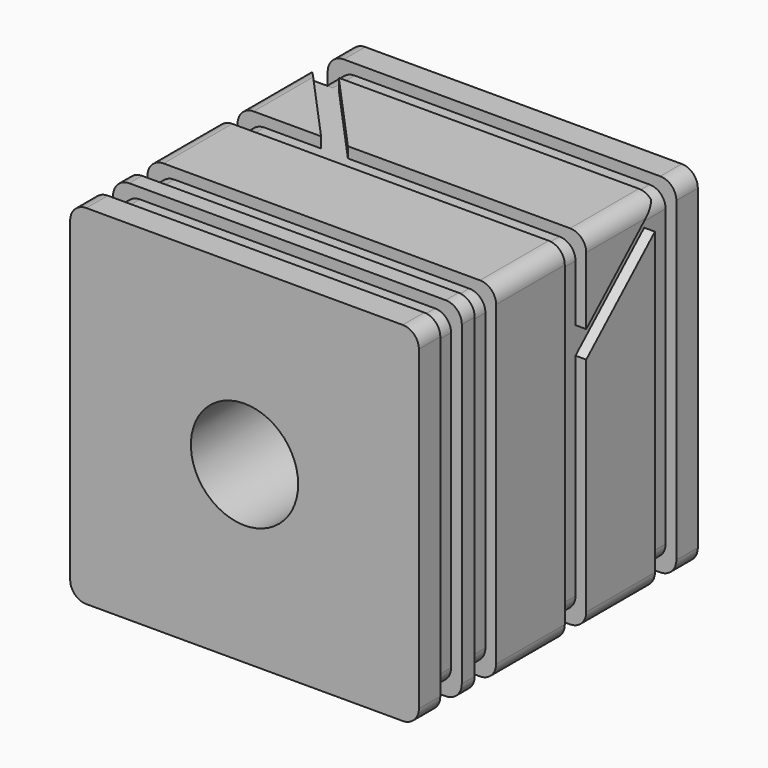
from build123d import *

# Parameters (mm, degrees)
F0_W      = 6.5
F0_H      = 6.5
F1_DEPTH  = 6.5
F2_R      = 1
F3_DEPTH  = 25
F4_W      = 0.5
F4_H      = 6.5
F5_DEPTH  = 0.2
F6_W      = 6.3
F6_H      = 0.5
F7_DEPTH  = 0.2
F8_W      = 0.5
F8_H      = 6.3
F9_DEPTH  = 0.2
F10_W     = 6.1
F10_H     = 0.5
F11_DEPTH = 0.2
F12_R     = 0.3


with BuildPart() as f1:
    # F0 (on Front) → F1 (new body)
    with BuildSketch(Plane.XZ):
        with Locations((3.25, -3.25)):
            Rectangle(F0_W, F0_H)
    extrude(amount=F1_DEPTH)

    # F2 (on face) → F3 (cut)
    with BuildSketch(Plane.XZ.offset(6.5)):
        with Locations((3.25, -3.25)):
            Circle(F2_R)
    extrude(amount=-F3_DEPTH, mode=Mode.SUBTRACT)

    # F4 (on face) → F5 (cut)
    with BuildSketch(Plane.YZ.offset(6.5)):
        with Locations((-5.75, -3.25)):
            Rectangle(F4_W, F4_H)
        with Locations((-4.95, -3.25)):
            Rectangle(F4_W, F4_H)
        Polygon((-3.1, 0), (-3.1, -6.5), (-2.6, -6.5), (-2.6, -2.0569080953), (-1, -0.6072367541), (-1, -6.5), (-0.5, -6.5), (-0.5, 0), (-1, 0), (-1, -0.1072367541), (-2.6, -1.5569080953), (-2.6, 0), align=None)
    extrude(amount=-F5_DEPTH, mode=Mode.SUBTRACT)

    # F6 (on face) → F7 (cut)
    with BuildSketch(Plane.XY):
        with Locations((3.15, -5.75)):
            Rectangle(F6_W, F6_H)
        with Locations((3.15, -4.95)):
            Rectangle(F6_W, F6_H)
        Polygon((0, -2.6), (0, -3.1), (6.3, -3.1), (6.3, -2.6), (2.0569080953, -2.6), (0.6072367541, -1), (6.3, -1), (6.3, -0.5), (0, -0.5), (0, -1), (0.1072367541, -1), (1.5569080953, -2.6), align=None)
    extrude(amount=-F7_DEPTH, mode=Mode.SUBTRACT)

    # F8 (on face) → F9 (cut)
    with BuildSketch(Plane(origin=(0, 0, 0), x_dir=(0, -1, 0), z_dir=(-1, 0, 0))):
        with Locations((5.75, -3.35)):
            Rectangle(F8_W, F8_H)
        with Locations((4.95, -3.35)):
            Rectangle(F8_W, F8_H)
        Polygon((2.6, -6.5), (3.1, -6.5), (3.1, -0.2), (2.6, -0.2), (2.6, -4.3532891255), (1, -5.8029604666), (1, -0.2), (0.5, -0.2), (0.5, -6.5), (1, -6.5), (1, -6.3029604666), (2.6, -4.8532891255), align=None)
    extrude(amount=-F9_DEPTH, mode=Mode.SUBTRACT)

    # F10 (on face) → F11 (cut)
    with BuildSketch(Plane(origin=(0, 0, -6.5), x_dir=(1, 0, 0), z_dir=(0, 0, -1))):
        with Locations((3.25, 5.75)):
            Rectangle(F10_W, F10_H)
        with Locations((3.25, 4.95)):
            Rectangle(F10_W, F10_H)
        Polygon((6.3, 3.1), (0.2, 3.1), (0.2, 2.6), (4.4430919047, 2.6), (5.8927632459, 1), (0.2, 1), (0.2, 0.5), (6.3, 0.5), (6.3, 1), (6.3927632459, 1), (4.9430919047, 2.6), (6.3, 2.6), align=None)
    extrude(amount=-F11_DEPTH, mode=Mode.SUBTRACT)

    # F12
    f12_edges = [f1.edges().sort_by_distance(p)[0] for p in [
        (0, -6.25, -6.5),
        (0.2, -5.75, -6.3),
        (0.2, -4.95, -6.3),
        (0, -5.35, -6.5),
        (0, -3.9, -6.5),
        (0.2, -2.85, -6.3),
        (0, -1.8, -6.5),
        (0.2, -0.75, -6.3),
        (0, -0.25, -6.5),
        (6.5, -0.25, -6.5),
        (6.3, -0.75, -6.3),
        (6.5, -1.8, -6.5),
        (6.3, -4.95, -6.3),
        (6.5, -3.9, -6.5),
        (6.5, -5.35, -6.5),
        (6.3, -5.75, -6.3),
        (6.5, -6.25, -6.5),
        (6.5, -0.25, 0),
        (6.3, -0.75, -0.2),
        (6.5, -1.8, 0),
        (6.3, -2.85, -0.2),
        (6.5, -3.9, 0),
        (6.3, -4.95, -0.2),
        (6.5, -5.35, 0),
        (6.3, -5.75, -0.2),
        (6.5, -6.25, 0),
        (0, -0.25, 0),
        (0.2, -0.75, -0.2),
        (0, -1.8, 0),
        (0.2, -2.85, -0.2),
        (0, -3.9, 0),
        (0.2, -4.95, -0.2),
        (0, -5.35, 0),
        (0.2, -5.75, -0.2),
        (0, -6.25, 0),
        (6.3, -2.85, -6.3),
    ]]
    fillet(f12_edges, radius=F12_R)


solid = f1.part
